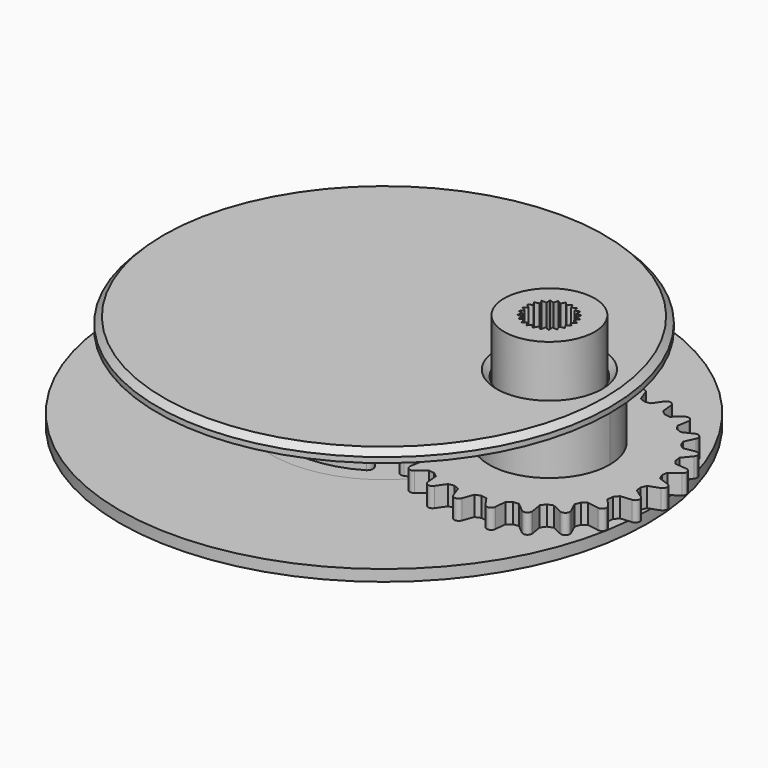
from build123d import *

# Parameters (mm, degrees)
F2_R       = 15
F3_DEPTH   = 1.5
F5_DEPTH   = 3
F6_R       = 4.2
F7_DEPTH   = 2.6
F9_R       = 4.1
F10_DEPTH  = 6.5
F11_SIZE2  = 6.49999
F11_SIZE   = 0.39999
F13_R      = 30
F13_R_2    = 6.2
F14_DEPTH  = 1.5
F15_R      = 6.3
F15_R_2    = 11.3
F16_DEPTH  = 7
F17_R      = 6.5
F18_DEPTH  = 7
F20_DEPTH  = 5
F21_R      = 6
F22_DEPTH  = 8
F23_SIZE   = 0.8
F23_2_SIZE = 0.8
F23_3_SIZE = 0.8
F25_DEPTH  = 3
F27_DEPTH  = 5
F28_SIZE   = 1


# Not quite as in the source:
# - a fillet or chamfer is up to 0.001 mm smaller than in the source, because OpenCascade refuses the exact size


with BuildPart() as f1:
    # F0 (on Front) → F1 (revolve)
    with BuildSketch(Plane.XZ):
        Polygon((0, 9), (0, 0), (35, 0), (35, 1.5), (8, 1.5), (8, 2.5), (4.2, 2.5), (3.8, 9), align=None)
    revolve(axis=Axis((0, 0, 4.5), (0, 0, 1)))


with BuildPart() as f3:
    # F2 (on Top) → F3 (new body)
    with BuildSketch(Plane.XY):
        Circle(F2_R)
    extrude(amount=F3_DEPTH)

    # F4 (on face) → F5 (join)
    with BuildSketch(Plane.XY.offset(1.5)):
        with BuildLine():
            ThreePointArc((6.1294095226, -0.4829629131), (6.3966766701, -0.3043807145), (6.5, 0))
            ThreePointArc((6.5, 0), (6.3966766701, 0.3043807145), (6.1294095226, 0.4829629131))
            ThreePointArc((6.1294095226, 0.4829629131), (5.5, 0), (6.1294095226, -0.4829629131))
        make_face()
        with BuildLine():
            ThreePointArc((6.1294095226, -0.4829629131), (5.5, 0), (6.1294095226, 0.4829629131))
            Line((6.1294095226, 0.4829629131), (4.19755787, 1.0006010033))
            Line((4.19755787, 1.0006010033), (4.1590994684, 1.1144273438))
            Line((4.1590994684, 1.1144273438), (4.1354922509, 1.232233047))
            Line((4.1354922509, 1.232233047), (5.5497058133, 2.6464466094))
            ThreePointArc((5.5497058133, 2.6464466094), (4.7631397208, 2.75), (5.0667429002, 3.4829629131))
            Line((5.0667429002, 3.4829629131), (3.1348912476, 2.9653248229))
            Line((3.1348912476, 2.9653248229), (3.0446721246, 3.0446721246))
            Line((3.0446721246, 3.0446721246), (2.9653248229, 3.1348912476))
            Line((2.9653248229, 3.1348912476), (3.4829629131, 5.0667429002))
            ThreePointArc((3.4829629131, 5.0667429002), (2.75, 4.7631397208), (2.6464466094, 5.5497058133))
            Line((2.6464466094, 5.5497058133), (1.232233047, 4.1354922509))
            Line((1.232233047, 4.1354922509), (1.1144273438, 4.1590994684))
            Line((1.1144273438, 4.1590994684), (1.0006010033, 4.19755787))
            Line((1.0006010033, 4.19755787), (0.4829629131, 6.1294095226))
            ThreePointArc((0.4829629131, 6.1294095226), (0.4957224307, 6.0652630961), (0.5, 6))
            ThreePointArc((0.5, 6), (-0.0652630961, 5.5042775693), (-0.4829629131, 6.1294095226))
            Line((-0.4829629131, 6.1294095226), (-1.0006010033, 4.19755787))
            Line((-1.0006010033, 4.19755787), (-1.1144273438, 4.1590994684))
            Line((-1.1144273438, 4.1590994684), (-1.232233047, 4.1354922509))
            Line((-1.232233047, 4.1354922509), (-2.6464466094, 5.5497058133))
            ThreePointArc((-2.6464466094, 5.5497058133), (-2.5380602337, 5.3874941389), (-2.5, 5.1961524227))
            ThreePointArc((-2.5, 5.1961524227), (-2.9347369039, 4.700429992), (-3.4829629131, 5.0667429002))
            Line((-3.4829629131, 5.0667429002), (-2.9653248229, 3.1348912476))
            Line((-2.9653248229, 3.1348912476), (-3.0446721246, 3.0446721246))
            Line((-3.0446721246, 3.0446721246), (-3.1348912476, 2.9653248229))
            Line((-3.1348912476, 2.9653248229), (-5.0667429002, 3.4829629131))
            ThreePointArc((-5.0667429002, 3.4829629131), (-4.7994757526, 3.3043807145), (-4.6961524227, 3))
            ThreePointArc((-4.6961524227, 3), (-5.0048107065, 2.5380602337), (-5.5497058133, 2.6464466094))
            Line((-5.5497058133, 2.6464466094), (-4.1354922509, 1.232233047))
            Line((-4.1354922509, 1.232233047), (-4.1590994684, 1.1144273438))
            Line((-4.1590994684, 1.1144273438), (-4.19755787, 1.0006010033))
            Line((-4.19755787, 1.0006010033), (-6.1294095226, 0.4829629131))
            ThreePointArc((-6.1294095226, 0.4829629131), (-5.6956192855, 0.3966766701), (-5.5, 0))
            ThreePointArc((-5.5, 0), (-5.6956192855, -0.3966766701), (-6.1294095226, -0.4829629131))
            Line((-6.1294095226, -0.4829629131), (-4.19755787, -1.0006010033))
            Line((-4.19755787, -1.0006010033), (-4.1590994684, -1.1144273438))
            Line((-4.1590994684, -1.1144273438), (-4.1354922509, -1.232233047))
            Line((-4.1354922509, -1.232233047), (-5.5497058133, -2.6464466094))
            ThreePointArc((-5.5497058133, -2.6464466094), (-5.0048107065, -2.5380602337), (-4.6961524227, -3))
            ThreePointArc((-4.6961524227, -3), (-4.7994757526, -3.3043807145), (-5.0667429002, -3.4829629131))
            Line((-5.0667429002, -3.4829629131), (-3.1348912476, -2.9653248229))
            Line((-3.1348912476, -2.9653248229), (-3.0446721246, -3.0446721246))
            Line((-3.0446721246, -3.0446721246), (-2.9653248229, -3.1348912476))
            Line((-2.9653248229, -3.1348912476), (-3.4829629131, -5.0667429002))
            ThreePointArc((-3.4829629131, -5.0667429002), (-2.9347369039, -4.700429992), (-2.5, -5.1961524227))
            ThreePointArc((-2.5, -5.1961524227), (-2.5380602337, -5.3874941389), (-2.6464466094, -5.5497058133))
            Line((-2.6464466094, -5.5497058133), (-1.232233047, -4.1354922509))
            Line((-1.232233047, -4.1354922509), (-1.1144273438, -4.1590994684))
            Line((-1.1144273438, -4.1590994684), (-1.0006010033, -4.19755787))
            Line((-1.0006010033, -4.19755787), (-0.4829629131, -6.1294095226))
            ThreePointArc((-0.4829629131, -6.1294095226), (-0.0652630961, -5.5042775693), (0.5, -6))
            ThreePointArc((0.5, -6), (0.4957224307, -6.0652630961), (0.4829629131, -6.1294095226))
            Line((0.4829629131, -6.1294095226), (1.0006010033, -4.19755787))
            Line((1.0006010033, -4.19755787), (1.1144273438, -4.1590994684))
            Line((1.1144273438, -4.1590994684), (1.232233047, -4.1354922509))
            Line((1.232233047, -4.1354922509), (2.6464466094, -5.5497058133))
            ThreePointArc((2.6464466094, -5.5497058133), (2.75, -4.7631397208), (3.4829629131, -5.0667429002))
            Line((3.4829629131, -5.0667429002), (2.9653248229, -3.1348912476))
            Line((2.9653248229, -3.1348912476), (3.0446721246, -3.0446721246))
            Line((3.0446721246, -3.0446721246), (3.1348912476, -2.9653248229))
            Line((3.1348912476, -2.9653248229), (5.0667429002, -3.4829629131))
            ThreePointArc((5.0667429002, -3.4829629131), (4.7631397208, -2.75), (5.5497058133, -2.6464466094))
            Line((5.5497058133, -2.6464466094), (4.1354922509, -1.232233047))
            Line((4.1354922509, -1.232233047), (4.1590994684, -1.1144273438))
            Line((4.1590994684, -1.1144273438), (4.19755787, -1.0006010033))
            Line((4.19755787, -1.0006010033), (6.1294095226, -0.4829629131))
        make_face()
        with BuildLine():
            ThreePointArc((5.0667429002, 3.4829629131), (4.7631397208, 2.75), (5.5497058133, 2.6464466094))
            ThreePointArc((5.5497058133, 2.6464466094), (5.658092189, 2.8086582838), (5.6961524227, 3))
            ThreePointArc((5.6961524227, 3), (5.5005331372, 3.3966766701), (5.0667429002, 3.4829629131))
        make_face()
        with BuildLine():
            ThreePointArc((5.6961524227, -3), (5.658092189, -2.8086582838), (5.5497058133, -2.6464466094))
            ThreePointArc((5.5497058133, -2.6464466094), (4.7631397208, -2.75), (5.0667429002, -3.4829629131))
            ThreePointArc((5.0667429002, -3.4829629131), (5.5005331372, -3.3966766701), (5.6961524227, -3))
        make_face()
        with BuildLine():
            ThreePointArc((2.6464466094, 5.5497058133), (2.75, 4.7631397208), (3.4829629131, 5.0667429002))
            ThreePointArc((3.4829629131, 5.0667429002), (3.4957224307, 5.1308893266), (3.5, 5.1961524227))
            ThreePointArc((3.5, 5.1961524227), (3.1913417162, 5.658092189), (2.6464466094, 5.5497058133))
        make_face()
        with BuildLine():
            ThreePointArc((3.5, -5.1961524227), (3.4957224307, -5.1308893266), (3.4829629131, -5.0667429002))
            ThreePointArc((3.4829629131, -5.0667429002), (2.75, -4.7631397208), (2.6464466094, -5.5497058133))
            ThreePointArc((2.6464466094, -5.5497058133), (3.1913417162, -5.658092189), (3.5, -5.1961524227))
        make_face()
        with BuildLine():
            ThreePointArc((0.5, 6), (0.4957224307, 6.0652630961), (0.4829629131, 6.1294095226))
            ThreePointArc((0.4829629131, 6.1294095226), (0, 6.5), (-0.4829629131, 6.1294095226))
            ThreePointArc((-0.4829629131, 6.1294095226), (-0.0652630961, 5.5042775693), (0.5, 6))
        make_face()
        with BuildLine():
            ThreePointArc((-0.4829629131, -6.1294095226), (0, -6.5), (0.4829629131, -6.1294095226))
            ThreePointArc((0.4829629131, -6.1294095226), (0.4957224307, -6.0652630961), (0.5, -6))
            ThreePointArc((0.5, -6), (-0.0652630961, -5.5042775693), (-0.4829629131, -6.1294095226))
        make_face()
        with BuildLine():
            ThreePointArc((-2.5, 5.1961524227), (-2.5380602337, 5.3874941389), (-2.6464466094, 5.5497058133))
            ThreePointArc((-2.6464466094, 5.5497058133), (-3.25, 5.6291651246), (-3.4829629131, 5.0667429002))
            ThreePointArc((-3.4829629131, 5.0667429002), (-2.9347369039, 4.700429992), (-2.5, 5.1961524227))
        make_face()
        with BuildLine():
            ThreePointArc((-3.4829629131, -5.0667429002), (-3.25, -5.6291651246), (-2.6464466094, -5.5497058133))
            ThreePointArc((-2.6464466094, -5.5497058133), (-2.5380602337, -5.3874941389), (-2.5, -5.1961524227))
            ThreePointArc((-2.5, -5.1961524227), (-2.9347369039, -4.700429992), (-3.4829629131, -5.0667429002))
        make_face()
        with BuildLine():
            ThreePointArc((-4.6961524227, 3), (-4.7994757526, 3.3043807145), (-5.0667429002, 3.4829629131))
            ThreePointArc((-5.0667429002, 3.4829629131), (-5.6291651246, 3.25), (-5.5497058133, 2.6464466094))
            ThreePointArc((-5.5497058133, 2.6464466094), (-5.0048107065, 2.5380602337), (-4.6961524227, 3))
        make_face()
        with BuildLine():
            ThreePointArc((-5.5497058133, -2.6464466094), (-5.6291651246, -3.25), (-5.0667429002, -3.4829629131))
            ThreePointArc((-5.0667429002, -3.4829629131), (-4.7994757526, -3.3043807145), (-4.6961524227, -3))
            ThreePointArc((-4.6961524227, -3), (-5.0048107065, -2.5380602337), (-5.5497058133, -2.6464466094))
        make_face()
        with BuildLine():
            ThreePointArc((-5.5, 0), (-5.6956192855, 0.3966766701), (-6.1294095226, 0.4829629131))
            ThreePointArc((-6.1294095226, 0.4829629131), (-6.5, 0), (-6.1294095226, -0.4829629131))
            ThreePointArc((-6.1294095226, -0.4829629131), (-5.6956192855, -0.3966766701), (-5.5, 0))
        make_face()
    extrude(amount=F5_DEPTH)

    # F9 (on face) → F10 (join)
    with BuildSketch(Plane.XY.offset(4.5)):
        Circle(F9_R)
    extrude(amount=F10_DEPTH)

    # F11 (size 0.4 and 6.5 in the source; OpenCascade refuses exactly that, so slightly less here)
    f11_edges = [f3.edges().sort_by_distance(p)[0] for p in [
        (-4.1, 0, 11),
    ]]
    f11_side = f3.faces().sort_by_distance((0, 0, 11))[0]
    chamfer(f11_edges, length=F11_SIZE, length2=F11_SIZE2, reference=f11_side)


with BuildPart() as f7:
    # F6 (on face) → F7 (new body)
    with BuildSketch(Plane.XY.offset(1.5)):
        with BuildLine():
            ThreePointArc((36.005212086, 0.8361844275), (36.2914912266, 1.0558541382), (36.4, 1.4))
            ThreePointArc((36.4, 1.4), (36.2914912266, 1.7441458618), (36.005212086, 1.9638155725))
            ThreePointArc((36.005212086, 1.9638155725), (35.2, 1.4), (36.005212086, 0.8361844275))
        make_face()
        with BuildLine():
            ThreePointArc((36.005212086, 0.8361844275), (35.2, 1.4), (36.005212086, 1.9638155725))
            Line((36.005212086, 1.9638155725), (34.5956731548, 2.4768457875))
            Line((34.5956731548, 2.4768457875), (34.2894922687, 3.1759253484))
            Line((34.2894922687, 3.1759253484), (34.4043051897, 3.9304297954))
            Line((34.4043051897, 3.9304297954), (35.6330332561, 4.79079445))
            ThreePointArc((35.6330332561, 4.79079445), (34.7093318986, 5.1269942495), (35.34118084, 5.8800024954))
            Line((35.34118084, 5.8800024954), (33.8468887928, 6.0107361095))
            Line((33.8468887928, 6.0107361095), (33.3702056631, 6.6067496675))
            Line((33.3702056631, 6.6067496675), (33.2858263081, 7.3652607695))
            Line((33.2858263081, 7.3652607695), (34.2500077226, 8.5143274342))
            ThreePointArc((34.2500077226, 8.5143274342), (33.2707658145, 8.6), (33.6861921502, 9.4908846518))
            Line((33.6861921502, 9.4908846518), (32.2089805206, 9.2304123853))
            Line((32.2089805206, 9.2304123853), (31.5942803147, 9.6827426013))
            Line((31.5942803147, 9.6827426013), (31.3164589974, 10.3935690802))
            Line((31.3164589974, 10.3935690802), (31.95038639, 11.7530307608))
            ThreePointArc((31.95038639, 11.7530307608), (30.9823376491, 11.5823376491), (31.1530307608, 12.55038639))
            Line((31.1530307608, 12.55038639), (29.7935690802, 11.9164589974))
            Line((29.7935690802, 11.9164589974), (29.0827426013, 12.1942803147))
            Line((29.0827426013, 12.1942803147), (28.6304123853, 12.8089805206))
            Line((28.6304123853, 12.8089805206), (28.8908846518, 14.2861921502))
            ThreePointArc((28.8908846518, 14.2861921502), (28, 13.8707658145), (27.9143274342, 14.8500077226))
            Line((27.9143274342, 14.8500077226), (26.7652607695, 13.8858263081))
            Line((26.7652607695, 13.8858263081), (26.0067496675, 13.9702056631))
            Line((26.0067496675, 13.9702056631), (25.4107361095, 14.4468887928))
            Line((25.4107361095, 14.4468887928), (25.2800024954, 15.94118084))
            ThreePointArc((25.2800024954, 15.94118084), (25.2817146095, 15.9150590268), (25.2822856765, 15.8888873943))
            ThreePointArc((25.2822856765, 15.8888873943), (24.5018621968, 15.3166572239), (24.19079445, 16.2330332561))
            Line((24.19079445, 16.2330332561), (23.3304297954, 15.0043051897))
            Line((23.3304297954, 15.0043051897), (22.5759253484, 14.8894922687))
            Line((22.5759253484, 14.8894922687), (21.8768457875, 15.1956731548))
            Line((21.8768457875, 15.1956731548), (21.3638155725, 16.605212086))
            ThreePointArc((21.3638155725, 16.605212086), (21.3908846518, 16.5041889066), (21.4, 16.4))
            ThreePointArc((21.4, 16.4), (20.6958110934, 15.8091153482), (20.2361844275, 16.605212086))
            Line((20.2361844275, 16.605212086), (19.7231542125, 15.1956731548))
            Line((19.7231542125, 15.1956731548), (19.0240746516, 14.8894922687))
            Line((19.0240746516, 14.8894922687), (18.2695702046, 15.0043051897))
            Line((18.2695702046, 15.0043051897), (17.40920555, 16.2330332561))
            ThreePointArc((17.40920555, 16.2330332561), (17.4899444939, 16.069310874), (17.5177143235, 15.8888873943))
            ThreePointArc((17.5177143235, 15.8888873943), (16.891542691, 15.2894584614), (16.3199975046, 15.94118084))
            Line((16.3199975046, 15.94118084), (16.1892638905, 14.4468887928))
            Line((16.1892638905, 14.4468887928), (15.5932503325, 13.9702056631))
            Line((15.5932503325, 13.9702056631), (14.8347392305, 13.8858263081))
            Line((14.8347392305, 13.8858263081), (13.6856725658, 14.8500077226))
            ThreePointArc((13.6856725658, 14.8500077226), (13.8437846722, 14.6439520138), (13.9, 14.3903810568))
            ThreePointArc((13.9, 14.3903810568), (13.3522934456, 13.7926642379), (12.7091153482, 14.2861921502))
            Line((12.7091153482, 14.2861921502), (12.9695876147, 12.8089805206))
            Line((12.9695876147, 12.8089805206), (12.5172573987, 12.1942803147))
            Line((12.5172573987, 12.1942803147), (11.8064309198, 11.9164589974))
            Line((11.8064309198, 11.9164589974), (10.4469692392, 12.55038639))
            ThreePointArc((10.4469692392, 12.55038639), (10.6994331497, 12.3289814828), (10.7933982822, 12.0066017178))
            ThreePointArc((10.7933982822, 12.0066017178), (10.3232620506, 11.4208241135), (9.64961361, 11.7530307608))
            Line((9.64961361, 11.7530307608), (10.2835410026, 10.3935690802))
            Line((10.2835410026, 10.3935690802), (10.0057196853, 9.6827426013))
            Line((10.0057196853, 9.6827426013), (9.3910194794, 9.2304123853))
            Line((9.3910194794, 9.2304123853), (7.9138078498, 9.4908846518))
            ThreePointArc((7.9138078498, 9.4908846518), (8.2692456091, 9.2856725658), (8.4096189432, 8.9))
            ThreePointArc((8.4096189432, 8.9), (8.0148310292, 8.3361844275), (7.3499922774, 8.5143274342))
            Line((7.3499922774, 8.5143274342), (8.3141736919, 7.3652607695))
            Line((8.3141736919, 7.3652607695), (8.2297943369, 6.6067496675))
            Line((8.2297943369, 6.6067496675), (7.7531112072, 6.0107361095))
            Line((7.7531112072, 6.0107361095), (6.25881916, 5.8800024954))
            ThreePointArc((6.25881916, 5.8800024954), (6.7164667302, 5.7246520786), (6.9111126057, 5.2822856765))
            ThreePointArc((6.9111126057, 5.2822856765), (6.5881617736, 4.7500791766), (5.9669667439, 4.79079445))
            Line((5.9669667439, 4.79079445), (7.1956948103, 3.9304297954))
            Line((7.1956948103, 3.9304297954), (7.3105077313, 3.1759253484))
            Line((7.3105077313, 3.1759253484), (7.0043268452, 2.4768457875))
            Line((7.0043268452, 2.4768457875), (5.594787914, 1.9638155725))
            ThreePointArc((5.594787914, 1.9638155725), (6.1441458618, 1.8914912266), (6.4, 1.4))
            ThreePointArc((6.4, 1.4), (6.1441458618, 0.9085087734), (5.594787914, 0.8361844275))
            Line((5.594787914, 0.8361844275), (7.0043268452, 0.3231542125))
            Line((7.0043268452, 0.3231542125), (7.3105077313, -0.3759253484))
            Line((7.3105077313, -0.3759253484), (7.1956948103, -1.1304297954))
            Line((7.1956948103, -1.1304297954), (5.9669667439, -1.99079445))
            ThreePointArc((5.9669667439, -1.99079445), (6.5881617736, -1.9500791766), (6.9111126057, -2.4822856765))
            ThreePointArc((6.9111126057, -2.4822856765), (6.7164667302, -2.9246520786), (6.25881916, -3.0800024954))
            Line((6.25881916, -3.0800024954), (7.7531112072, -3.2107361095))
            Line((7.7531112072, -3.2107361095), (8.2297943369, -3.8067496675))
            Line((8.2297943369, -3.8067496675), (8.3141736919, -4.5652607695))
            Line((8.3141736919, -4.5652607695), (7.3499922774, -5.7143274342))
            ThreePointArc((7.3499922774, -5.7143274342), (8.0148310292, -5.5361844275), (8.4096189432, -6.1))
            ThreePointArc((8.4096189432, -6.1), (8.2692456091, -6.4856725658), (7.9138078498, -6.6908846518))
            Line((7.9138078498, -6.6908846518), (9.3910194794, -6.4304123853))
            Line((9.3910194794, -6.4304123853), (10.0057196853, -6.8827426013))
            Line((10.0057196853, -6.8827426013), (10.2835410026, -7.5935690802))
            Line((10.2835410026, -7.5935690802), (9.64961361, -8.9530307608))
            ThreePointArc((9.64961361, -8.9530307608), (10.3232620506, -8.6208241135), (10.7933982822, -9.2066017178))
            ThreePointArc((10.7933982822, -9.2066017178), (10.6994331497, -9.5289814828), (10.4469692392, -9.75038639))
            Line((10.4469692392, -9.75038639), (11.8064309198, -9.1164589974))
            Line((11.8064309198, -9.1164589974), (12.5172573987, -9.3942803147))
            Line((12.5172573987, -9.3942803147), (12.9695876147, -10.0089805206))
            Line((12.9695876147, -10.0089805206), (12.7091153482, -11.4861921502))
            ThreePointArc((12.7091153482, -11.4861921502), (13.3522934456, -10.9926642379), (13.9, -11.5903810568))
            ThreePointArc((13.9, -11.5903810568), (13.8437846722, -11.8439520138), (13.6856725658, -12.0500077226))
            Line((13.6856725658, -12.0500077226), (14.8347392305, -11.0858263081))
            Line((14.8347392305, -11.0858263081), (15.5932503325, -11.1702056631))
            Line((15.5932503325, -11.1702056631), (16.1892638905, -11.6468887928))
            Line((16.1892638905, -11.6468887928), (16.3199975046, -13.14118084))
            ThreePointArc((16.3199975046, -13.14118084), (16.891542691, -12.4894584614), (17.5177143235, -13.0888873943))
            ThreePointArc((17.5177143235, -13.0888873943), (17.4899444939, -13.269310874), (17.40920555, -13.4330332561))
            Line((17.40920555, -13.4330332561), (18.2695702046, -12.2043051897))
            Line((18.2695702046, -12.2043051897), (19.0240746516, -12.0894922687))
            Line((19.0240746516, -12.0894922687), (19.7231542125, -12.3956731548))
            Line((19.7231542125, -12.3956731548), (20.2361844275, -13.805212086))
            ThreePointArc((20.2361844275, -13.805212086), (20.6958110934, -13.0091153482), (21.4, -13.6))
            ThreePointArc((21.4, -13.6), (21.3908846518, -13.7041889066), (21.3638155725, -13.805212086))
            Line((21.3638155725, -13.805212086), (21.8768457875, -12.3956731548))
            Line((21.8768457875, -12.3956731548), (22.5759253484, -12.0894922687))
            Line((22.5759253484, -12.0894922687), (23.3304297954, -12.2043051897))
            Line((23.3304297954, -12.2043051897), (24.19079445, -13.4330332561))
            ThreePointArc((24.19079445, -13.4330332561), (24.5018621968, -12.5166572239), (25.2822856765, -13.0888873943))
            ThreePointArc((25.2822856765, -13.0888873943), (25.2817146095, -13.1150590268), (25.2800024954, -13.14118084))
            Line((25.2800024954, -13.14118084), (25.4107361095, -11.6468887928))
            Line((25.4107361095, -11.6468887928), (26.0067496675, -11.1702056631))
            Line((26.0067496675, -11.1702056631), (26.7652607695, -11.0858263081))
            Line((26.7652607695, -11.0858263081), (27.9143274342, -12.0500077226))
            ThreePointArc((27.9143274342, -12.0500077226), (28, -11.0707658145), (28.8908846518, -11.4861921502))
            Line((28.8908846518, -11.4861921502), (28.6304123853, -10.0089805206))
            Line((28.6304123853, -10.0089805206), (29.0827426013, -9.3942803147))
            Line((29.0827426013, -9.3942803147), (29.7935690802, -9.1164589974))
            Line((29.7935690802, -9.1164589974), (31.1530307608, -9.75038639))
            ThreePointArc((31.1530307608, -9.75038639), (30.9823376491, -8.7823376491), (31.95038639, -8.9530307608))
            Line((31.95038639, -8.9530307608), (31.3164589974, -7.5935690802))
            Line((31.3164589974, -7.5935690802), (31.5942803147, -6.8827426013))
            Line((31.5942803147, -6.8827426013), (32.2089805206, -6.4304123853))
            Line((32.2089805206, -6.4304123853), (33.6861921502, -6.6908846518))
            ThreePointArc((33.6861921502, -6.6908846518), (33.2707658145, -5.8), (34.2500077226, -5.7143274342))
            Line((34.2500077226, -5.7143274342), (33.2858263081, -4.5652607695))
            Line((33.2858263081, -4.5652607695), (33.3702056631, -3.8067496675))
            Line((33.3702056631, -3.8067496675), (33.8468887928, -3.2107361095))
            Line((33.8468887928, -3.2107361095), (35.34118084, -3.0800024954))
            ThreePointArc((35.34118084, -3.0800024954), (34.7093318986, -2.3269942495), (35.6330332561, -1.99079445))
            Line((35.6330332561, -1.99079445), (34.4043051897, -1.1304297954))
            Line((34.4043051897, -1.1304297954), (34.2894922687, -0.3759253484))
            Line((34.2894922687, -0.3759253484), (34.5956731548, 0.3231542125))
            Line((34.5956731548, 0.3231542125), (36.005212086, 0.8361844275))
        make_face()
        with Locations((20.8, 1.4)):
            Circle(F6_R, mode=Mode.SUBTRACT)
        with BuildLine():
            ThreePointArc((35.34118084, 5.8800024954), (34.7093318986, 5.1269942495), (35.6330332561, 4.79079445))
            ThreePointArc((35.6330332561, 4.79079445), (35.8210938942, 5.0052365086), (35.8888873943, 5.2822856765))
            ThreePointArc((35.8888873943, 5.2822856765), (35.7312537964, 5.6876398011), (35.34118084, 5.8800024954))
        make_face()
        with BuildLine():
            ThreePointArc((35.8888873943, -2.4822856765), (35.8210938942, -2.2052365086), (35.6330332561, -1.99079445))
            ThreePointArc((35.6330332561, -1.99079445), (34.7093318986, -2.3269942495), (35.34118084, -3.0800024954))
            ThreePointArc((35.34118084, -3.0800024954), (35.7312537964, -2.8876398011), (35.8888873943, -2.4822856765))
        make_face()
        with BuildLine():
            ThreePointArc((33.6861921502, 9.4908846518), (33.2707658145, 8.6), (34.2500077226, 8.5143274342))
            ThreePointArc((34.2500077226, 8.5143274342), (34.3541966292, 8.694787914), (34.3903810568, 8.9))
            ThreePointArc((34.3903810568, 8.9), (34.1760536226, 9.3596266659), (33.6861921502, 9.4908846518))
        make_face()
        with BuildLine():
            ThreePointArc((34.3903810568, -6.1), (34.3541966292, -5.894787914), (34.2500077226, -5.7143274342))
            ThreePointArc((34.2500077226, -5.7143274342), (33.2707658145, -5.8), (33.6861921502, -6.6908846518))
            ThreePointArc((33.6861921502, -6.6908846518), (34.1760536226, -6.5596266659), (34.3903810568, -6.1))
        make_face()
        with BuildLine():
            ThreePointArc((31.1530307608, 12.55038639), (30.9823376491, 11.5823376491), (31.95038639, 11.7530307608))
            ThreePointArc((31.95038639, 11.7530307608), (31.9923793221, 11.8767379494), (32.0066017178, 12.0066017178))
            ThreePointArc((32.0066017178, 12.0066017178), (31.7289814828, 12.5126365853), (31.1530307608, 12.55038639))
        make_face()
        with BuildLine():
            ThreePointArc((32.0066017178, -9.2066017178), (31.9923793221, -9.0767379494), (31.95038639, -8.9530307608))
            ThreePointArc((31.95038639, -8.9530307608), (30.9823376491, -8.7823376491), (31.1530307608, -9.75038639))
            ThreePointArc((31.1530307608, -9.75038639), (31.7289814828, -9.7126365853), (32.0066017178, -9.2066017178))
        make_face()
        with BuildLine():
            ThreePointArc((27.9143274342, 14.8500077226), (28, 13.8707658145), (28.8908846518, 14.2861921502))
            ThreePointArc((28.8908846518, 14.2861921502), (28.8977168189, 14.3380876111), (28.9, 14.3903810568))
            ThreePointArc((28.9, 14.3903810568), (28.553570957, 14.934165729), (27.9143274342, 14.8500077226))
        make_face()
        with BuildLine():
            ThreePointArc((28.9, -11.5903810568), (28.8977168189, -11.5380876111), (28.8908846518, -11.4861921502))
            ThreePointArc((28.8908846518, -11.4861921502), (28, -11.0707658145), (27.9143274342, -12.0500077226))
            ThreePointArc((27.9143274342, -12.0500077226), (28.553570957, -12.134165729), (28.9, -11.5903810568))
        make_face()
        with BuildLine():
            ThreePointArc((25.2822856765, 15.8888873943), (25.2817146095, 15.9150590268), (25.2800024954, 15.94118084))
            ThreePointArc((25.2800024954, 15.94118084), (24.8375771036, 16.4684428901), (24.19079445, 16.2330332561))
            ThreePointArc((24.19079445, 16.2330332561), (24.5018621968, 15.3166572239), (25.2822856765, 15.8888873943))
        make_face()
        with BuildLine():
            ThreePointArc((24.19079445, -13.4330332561), (24.8375771036, -13.6684428901), (25.2800024954, -13.14118084))
            ThreePointArc((25.2800024954, -13.14118084), (25.2817146095, -13.1150590268), (25.2822856765, -13.0888873943))
            ThreePointArc((25.2822856765, -13.0888873943), (24.5018621968, -12.5166572239), (24.19079445, -13.4330332561))
        make_face()
        with BuildLine():
            ThreePointArc((21.4, 16.4), (21.3908846518, 16.5041889066), (21.3638155725, 16.605212086))
            ThreePointArc((21.3638155725, 16.605212086), (20.8, 17), (20.2361844275, 16.605212086))
            ThreePointArc((20.2361844275, 16.605212086), (20.6958110934, 15.8091153482), (21.4, 16.4))
        make_face()
        with BuildLine():
            ThreePointArc((20.2361844275, -13.805212086), (20.8, -14.2), (21.3638155725, -13.805212086))
            ThreePointArc((21.3638155725, -13.805212086), (21.3908846518, -13.7041889066), (21.4, -13.6))
            ThreePointArc((21.4, -13.6), (20.6958110934, -13.0091153482), (20.2361844275, -13.805212086))
        make_face()
        with BuildLine():
            ThreePointArc((17.5177143235, 15.8888873943), (17.4899444939, 16.069310874), (17.40920555, 16.2330332561))
            ThreePointArc((17.40920555, 16.2330332561), (16.7624228964, 16.4684428901), (16.3199975046, 15.94118084))
            ThreePointArc((16.3199975046, 15.94118084), (16.891542691, 15.2894584614), (17.5177143235, 15.8888873943))
        make_face()
        with BuildLine():
            ThreePointArc((16.3199975046, -13.14118084), (16.7624228964, -13.6684428901), (17.40920555, -13.4330332561))
            ThreePointArc((17.40920555, -13.4330332561), (17.4899444939, -13.269310874), (17.5177143235, -13.0888873943))
            ThreePointArc((17.5177143235, -13.0888873943), (16.891542691, -12.4894584614), (16.3199975046, -13.14118084))
        make_face()
        with BuildLine():
            ThreePointArc((13.9, 14.3903810568), (13.8437846722, 14.6439520138), (13.6856725658, 14.8500077226))
            ThreePointArc((13.6856725658, 14.8500077226), (13, 14.909996299), (12.7091153482, 14.2861921502))
            ThreePointArc((12.7091153482, 14.2861921502), (13.3522934456, 13.7926642379), (13.9, 14.3903810568))
        make_face()
        with BuildLine():
            ThreePointArc((12.7091153482, -11.4861921502), (13, -12.109996299), (13.6856725658, -12.0500077226))
            ThreePointArc((13.6856725658, -12.0500077226), (13.8437846722, -11.8439520138), (13.9, -11.5903810568))
            ThreePointArc((13.9, -11.5903810568), (13.3522934456, -10.9926642379), (12.7091153482, -11.4861921502))
        make_face()
        with BuildLine():
            ThreePointArc((10.7933982822, 12.0066017178), (10.6994331497, 12.3289814828), (10.4469692392, 12.55038639))
            ThreePointArc((10.4469692392, 12.55038639), (9.7691342135, 12.4308657865), (9.64961361, 11.7530307608))
            ThreePointArc((9.64961361, 11.7530307608), (10.3232620506, 11.4208241135), (10.7933982822, 12.0066017178))
        make_face()
        with BuildLine():
            ThreePointArc((9.64961361, -8.9530307608), (9.7691342135, -9.6308657865), (10.4469692392, -9.75038639))
            ThreePointArc((10.4469692392, -9.75038639), (10.6994331497, -9.5289814828), (10.7933982822, -9.2066017178))
            ThreePointArc((10.7933982822, -9.2066017178), (10.3232620506, -8.6208241135), (9.64961361, -8.9530307608))
        make_face()
        with BuildLine():
            ThreePointArc((8.4096189432, 8.9), (8.2692456091, 9.2856725658), (7.9138078498, 9.4908846518))
            ThreePointArc((7.9138078498, 9.4908846518), (7.290003701, 9.2), (7.3499922774, 8.5143274342))
            ThreePointArc((7.3499922774, 8.5143274342), (8.0148310292, 8.3361844275), (8.4096189432, 8.9))
        make_face()
        with BuildLine():
            ThreePointArc((7.3499922774, -5.7143274342), (7.290003701, -6.4), (7.9138078498, -6.6908846518))
            ThreePointArc((7.9138078498, -6.6908846518), (8.2692456091, -6.4856725658), (8.4096189432, -6.1))
            ThreePointArc((8.4096189432, -6.1), (8.0148310292, -5.5361844275), (7.3499922774, -5.7143274342))
        make_face()
        with BuildLine():
            ThreePointArc((6.9111126057, 5.2822856765), (6.7164667302, 5.7246520786), (6.25881916, 5.8800024954))
            ThreePointArc((6.25881916, 5.8800024954), (5.7315571099, 5.4375771036), (5.9669667439, 4.79079445))
            ThreePointArc((5.9669667439, 4.79079445), (6.5881617736, 4.7500791766), (6.9111126057, 5.2822856765))
        make_face()
        with BuildLine():
            ThreePointArc((5.9669667439, -1.99079445), (5.7315571099, -2.6375771036), (6.25881916, -3.0800024954))
            ThreePointArc((6.25881916, -3.0800024954), (6.7164667302, -2.9246520786), (6.9111126057, -2.4822856765))
            ThreePointArc((6.9111126057, -2.4822856765), (6.5881617736, -1.9500791766), (5.9669667439, -1.99079445))
        make_face()
        with BuildLine():
            ThreePointArc((6.4, 1.4), (6.1441458618, 1.8914912266), (5.594787914, 1.9638155725))
            ThreePointArc((5.594787914, 1.9638155725), (5.2, 1.4), (5.594787914, 0.8361844275))
            ThreePointArc((5.594787914, 0.8361844275), (6.1441458618, 0.9085087734), (6.4, 1.4))
        make_face()
    extrude(amount=F7_DEPTH)

    # F17 (on face) → F18 (join)
    with BuildSketch(Plane.XY.offset(4.1)):
        with Locations((20.8, 1.4)):
            Circle(F17_R)
        Polygon((24.2, 3.2), (24.2, 1.4), (24.2, -0.4), (22.6, -0.4), (22.6, -2), (20.8, -2), (19, -2), (19, -0.4), (17.4, -0.4), (17.4, 1.4), (17.4, 3.2), (19, 3.2), (19, 4.8), (20.8, 4.8), (22.6, 4.8), (22.6, 3.2), align=None, mode=Mode.SUBTRACT)
    extrude(amount=F18_DEPTH)

    # F23
    f23_edges = [f7.edges().sort_by_distance(p)[0] for p in [
        (24.2, 1.4, 11.1),
        (23.4, -0.4, 11.1),
        (20.8, -2, 11.1),
        (22.6, -1.2, 11.1),
        (19, -1.2, 11.1),
        (18.2, -0.4, 11.1),
        (17.4, 1.4, 11.1),
        (18.2, 3.2, 11.1),
        (19, 4, 11.1),
        (20.8, 4.8, 11.1),
        (22.6, 4, 11.1),
        (23.4, 3.2, 11.1),
    ]]
    chamfer(f23_edges, length=F23_SIZE)


with BuildPart() as f14:
    # F13 (on offset) → F14 (new body)
    with BuildSketch(Plane.XY.offset(11.25)):
        Circle(F13_R)
        with Locations((20.8, 1.4)):
            Circle(F13_R_2, mode=Mode.SUBTRACT)
    extrude(amount=F14_DEPTH)

    # F15 (on face) → F16 (join)
    with BuildSketch(Plane(origin=(0, 0, 11.25), x_dir=(1, 0, 0), z_dir=(0, 0, -1))):
        with BuildLine():
            ThreePointArc((12.8301886792, -2.0943396226), (12.9574776255, -1.050606294), (13, 0))
            ThreePointArc((13, 0), (12.9987804306, 0.1780654854), (12.9951219512, 0.356097561))
            ThreePointArc((12.9951219512, 0.356097561), (12.8180599618, -0.8627540359), (12.8301886792, -2.0943396226))
        make_face()
        with BuildLine():
            ThreePointArc((12.9951219512, 0.356097561), (12.9987804306, 0.1780654854), (13, 0))
            ThreePointArc((13, 0), (12.9574776255, -1.050606294), (12.8301886792, -2.0943396226))
            ThreePointArc((12.8301886792, -2.0943396226), (21.1474977942, -9.3924492668), (28.8, -1.4))
            ThreePointArc((28.8, -1.4), (21.6834522086, 6.5510698774), (12.9951219512, 0.356097561))
        make_face()
        with Locations((20.8, -1.4)):
            Circle(F15_R, mode=Mode.SUBTRACT)
        with BuildLine():
            ThreePointArc((12.8301886792, -2.0943396226), (12.8180599618, -0.8627540359), (12.9951219512, 0.356097561))
            ThreePointArc((12.9951219512, 0.356097561), (-12.9706525621, 0.8730246917), (12.8301886792, -2.0943396226))
        make_face()
        Circle(F15_R_2, mode=Mode.SUBTRACT)
    extrude(amount=F16_DEPTH)

    # F23#2
    f23_2_edges = [f14.edges().sort_by_distance(p)[0] for p in [
        (-30, 0, 12.75),
        (14.6, 1.4, 12.75),
    ]]
    chamfer(f23_2_edges, length=F23_2_SIZE)

    # F24 (on face) → F25 (join)
    with BuildSketch(Plane(origin=(0, 0, 4.25), x_dir=(1, 0, 0), z_dir=(0, 0, -1))):
        with BuildLine():
            ThreePointArc((5.7036798817, 9.7548980419), (6.8238708368, 10.0475229439), (6.6212687523, 11.1874393902))
            ThreePointArc((6.6212687523, 11.1874393902), (-13, 0), (6.6212687523, -11.1874393902))
            ThreePointArc((6.6212687523, -11.1874393902), (6.8238708368, -10.0475229439), (5.7036798817, -9.7548980419))
            ThreePointArc((5.7036798817, -9.7548980419), (-11.3, 0), (5.7036798817, 9.7548980419))
        make_face()
    extrude(amount=F25_DEPTH)


with BuildPart() as f20:
    # F19 (on face) → F20 (new body)
    with BuildSketch(Plane.XY.offset(11.1)):
        Polygon((17.6, 1.4), (20.8, 1.4), (20.8, 4.6), (19.2, 4.6), (19.2, 3), (17.6, 3), align=None)
        Polygon((20.8, 4.6), (20.8, 1.4), (24, 1.4), (24, 3), (22.4, 3), (22.4, 4.6), align=None)
        Polygon((20.8, -1.8), (20.8, 1.4), (17.6, 1.4), (17.6, -0.2), (19.2, -0.2), (19.2, -1.8), align=None)
        Polygon((24, 1.4), (20.8, 1.4), (20.8, -1.8), (22.4, -1.8), (22.4, -0.2), (24, -0.2), align=None)
    extrude(amount=-F20_DEPTH)

    # F21 (on face) → F22 (join)
    with BuildSketch(Plane.XY.offset(11.1)):
        with Locations((20.8, 1.4)):
            Circle(F21_R)
    extrude(amount=F22_DEPTH)

    # F23#3
    f23_3_edges = [f20.edges().sort_by_distance(p)[0] for p in [
        (23.2, 3, 6.1),
        (22.4, 3.8, 6.1),
        (20.8, 4.6, 6.1),
        (19.2, 3.8, 6.1),
        (18.4, 3, 6.1),
        (17.6, 1.4, 6.1),
        (18.4, -0.2, 6.1),
        (19.2, -1, 6.1),
        (20.8, -1.8, 6.1),
        (22.4, -1, 6.1),
        (23.2, -0.2, 6.1),
        (24, 1.4, 6.1),
    ]]
    chamfer(f23_3_edges, length=F23_3_SIZE)

    # F26 (on face) → F27 (cut)
    with BuildSketch(Plane.XY.offset(19.1)):
        Polygon((24.0997422478, 0.9655806917), (23.6, 1.4), (24.0997422478, 1.8344193083), (23.5045923136, 2.1246933263), (23.8748702667, 2.673652967), (23.2248711306, 2.8), (23.4404509584, 3.4260892808), (22.7798989873, 3.3798989873), (22.8260892808, 4.0404509584), (22.2, 3.8248711306), (22.073652967, 4.4748702667), (21.5246933263, 4.1045923136), (21.2344193083, 4.6997422478), (20.8, 4.2), (20.3655806917, 4.6997422478), (20.0753066737, 4.1045923136), (19.526347033, 4.4748702667), (19.4, 3.8248711306), (18.7739107192, 4.0404509584), (18.8201010127, 3.3798989873), (18.1595490416, 3.4260892808), (18.3751288694, 2.8), (17.7251297333, 2.673652967), (18.0954076864, 2.1246933263), (17.5002577522, 1.8344193083), (18, 1.4), (17.5002577522, 0.9655806917), (18.0954076864, 0.6753066737), (17.7251297333, 0.126347033), (18.3751288694, 0), (18.1595490416, -0.6260892808), (18.8201010127, -0.5798989873), (18.7739107192, -1.2404509584), (19.4, -1.0248711306), (19.526347033, -1.6748702667), (20.0753066737, -1.3045923136), (20.3655806917, -1.8997422478), (20.8, -1.4), (21.2344193083, -1.8997422478), (21.5246933263, -1.3045923136), (22.073652967, -1.6748702667), (22.2, -1.0248711306), (22.8260892808, -1.2404509584), (22.7798989873, -0.5798989873), (23.4404509584, -0.6260892808), (23.2248711306, 0), (23.8748702667, 0.126347033), (23.5045923136, 0.6753066737), align=None)
    extrude(amount=-F27_DEPTH, mode=Mode.SUBTRACT)

    # F28
    f28_edges = [f20.edges().sort_by_distance(p)[0] for p in [
        (21.799173, -1.489731, 14.1),
        (22.136826, -1.349871, 14.1),
        (22.513045, -1.132661, 14.1),
        (22.802994, -0.910175, 14.1),
        (23.110175, -0.602994, 14.1),
        (23.332661, -0.313045, 14.1),
        (23.549871, 0.063174, 14.1),
        (23.689731, 0.400827, 14.1),
        (23.802167, 0.820444, 14.1),
        (23.849871, 1.18279, 14.1),
        (23.849871, 1.61721, 14.1),
        (23.802167, 1.979556, 14.1),
        (23.689731, 2.399173, 14.1),
        (23.549871, 2.736826, 14.1),
        (23.332661, 3.113045, 14.1),
        (23.110175, 3.402994, 14.1),
        (22.802994, 3.710175, 14.1),
        (22.513045, 3.932661, 14.1),
        (22.136826, 4.149871, 14.1),
        (21.799173, 4.289731, 14.1),
        (21.379556, 4.402167, 14.1),
        (21.01721, 4.449871, 14.1),
        (20.58279, 4.449871, 14.1),
        (20.220444, 4.402167, 14.1),
        (19.800827, 4.289731, 14.1),
        (19.463174, 4.149871, 14.1),
        (19.086955, 3.932661, 14.1),
        (18.797006, 3.710175, 14.1),
        (18.489825, 3.402994, 14.1),
        (18.267339, 3.113045, 14.1),
        (18.050129, 2.736826, 14.1),
        (17.910269, 2.399173, 14.1),
        (17.797833, 1.979556, 14.1),
        (17.750129, 1.61721, 14.1),
        (17.750129, 1.18279, 14.1),
        (17.797833, 0.820444, 14.1),
        (17.910269, 0.400827, 14.1),
        (18.050129, 0.063174, 14.1),
        (18.267339, -0.313045, 14.1),
        (18.489825, -0.602994, 14.1),
        (18.797006, -0.910175, 14.1),
        (19.086955, -1.132661, 14.1),
        (19.463174, -1.349871, 14.1),
        (19.800827, -1.489731, 14.1),
        (20.220444, -1.602167, 14.1),
        (20.58279, -1.649871, 14.1),
        (21.01721, -1.649871, 14.1),
        (21.379556, -1.602167, 14.1),
    ]]
    chamfer(f28_edges, length=F28_SIZE)


solid = Compound([f1.part, f3.part, f7.part, f14.part, f20.part])
